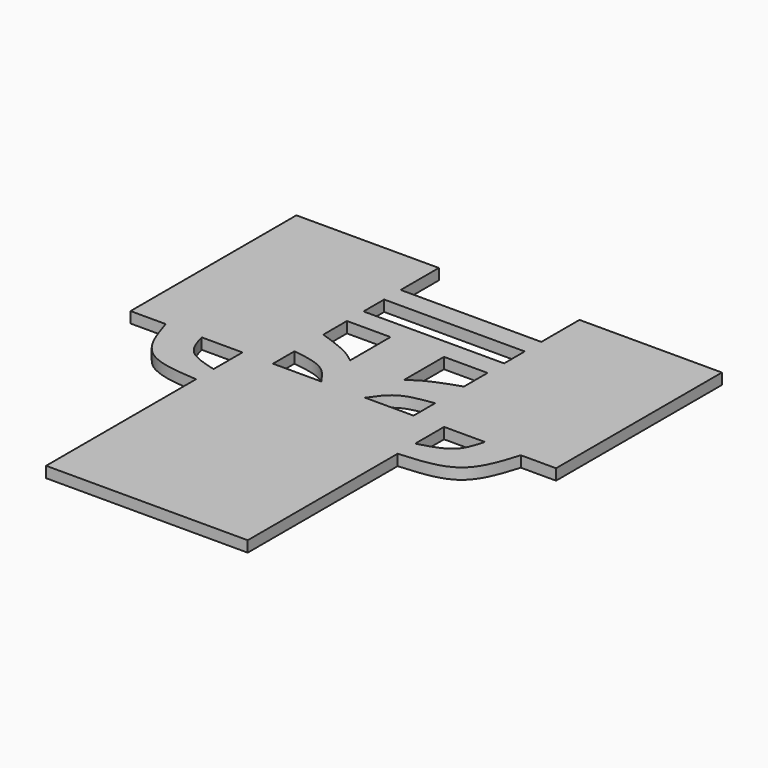
from build123d import *

# Parameters (mm, degrees)
F0_W     = 40.7416
F0_H     = 5.9913918376
F1_DEPTH = 3.175


# Not quite as in the source:
# - a feature names something its author has since deleted; it is built from what else it names


with BuildPart() as f1:
    # F0 (on Top) → F1 (new body)
    with BuildSketch(Plane.XY):
        Polygon((6.35, 2.420714612), (0, 2.420714612), (-6.35, 2.420714612), (-20.3708, 2.420714612), (-22.9107162118, 2.420714612), (-29.21, 2.420714612), (-29.21, -8.0478828564), (-29.21, -14.3978828564), (-29.21, -68.699285388), (29.21, -68.699285388), (29.21, -14.3978828564), (29.21, -8.0478828564), (29.21, 2.420714612), (20.3708, 2.420714612), align=None)
        Polygon((20.3708, 10.1967882365), (20.3708, 2.420714612), (29.21, 2.420714612), (41.0083, 2.420714612), (51.4477, 2.420714612), (61.6458, 2.420714612), (61.6458, 62.491714612), (20.3708, 62.491714612), (20.3708, 48.6805066466), (20.3708, 42.689114809), (20.3708, 35.2035965675), (20.3708, 29.2091965675), (20.3708, 20.6410996616), align=None)
        Polygon((-22.9107162118, 2.420714612), (-20.3708, 2.420714612), (-20.3708, 10.1967882365), (-20.3708, 20.6410996616), (-20.3708, 29.2091965675), (-20.3708, 35.2035965675), (-20.3708, 42.689114809), (-20.3708, 48.6805066466), (-20.3708, 62.491714612), (-61.6458, 62.491714612), (-61.6458, 2.420714612), (-51.4477, 2.420714612), (-41.0083, 2.420714612), (-29.21, 2.420714612), align=None)
        with BuildLine():
            add(Edge.make_bspline(
                [(29.21, -8.0478828564), (32.5638420451, -7.1347003919), (38.8822247108, -5.4143342635), (40.3293289084, -0.0814412218), (41.0083, 2.420714612)],
                knots=[0, 0, 0, 0, 0.5308070471, 1, 1, 1, 1], degree=3))
            Line((29.21, -8.0478828564), (29.21, -14.3978828564))
            add(Edge.make_bspline(
                [(29.21, -14.3978828564), (35.0623442189, -14.0006727781), (46.562333527, -13.2201459527), (49.8386841247, -2.7306682151), (51.4477, 2.420714612)],
                knots=[0, 0, 0, 0, 0.5088999704, 1, 1, 1, 1], degree=3))
            Line((51.4477, 2.420714612), (41.0083, 2.420714612))
        make_face()
        with BuildLine():
            Line((-29.21, -14.3978828564), (-29.21, -8.0478828564))
            add(Edge.make_bspline(
                [(-29.21, -8.0478828564), (-32.5638420451, -7.1347003919), (-38.8822247108, -5.4143342635), (-40.3293289084, -0.0814412218), (-41.0083, 2.420714612)],
                knots=[0, 0, 0, 0, 0.5308070471, 1, 1, 1, 1], degree=3))
            Line((-41.0083, 2.420714612), (-51.4477, 2.420714612))
            add(Edge.make_bspline(
                [(-29.21, -14.3978828564), (-35.0623442189, -14.0006727781), (-46.562333527, -13.2201459527), (-49.8386841247, -2.7306682151), (-51.4477, 2.420714612)],
                knots=[0, 0, 0, 0, 0.5088999704, 1, 1, 1, 1], degree=3))
        make_face()
        with Locations((0, 45.6848107278)):
            Rectangle(F0_W, F0_H)
        with BuildLine():
            Line((-6.35, 2.420714612), (0, 2.420714612))
            add(Edge.make_bspline(
                [(0, 2.420714612), (-2.1599363926, 6.9765171348), (-4.3198727852, 11.5323196577), (-7.7523121432, 14.5766604692)],
                knots=[0, 0, 0, 0, 0.5036722623, 0.5036722623, 0.5036722623, 0.5036722623], degree=3))
            add(Edge.make_bspline(
                [(-7.7523121432, 14.5766604692), (-11.1346998365, 17.5766088502), (-15.7527499182, 19.1088542559), (-20.3708, 20.6410996616)],
                knots=[0.5036722623, 0.5036722623, 0.5036722623, 0.5036722623, 1, 1, 1, 1], degree=3))
            Line((-20.3708, 20.6410996616), (-20.3708, 10.1967882365))
            add(Edge.make_bspline(
                [(-6.35, 2.420714612), (-7.7523121432, 4.4872624945), (-10.7420432518, 8.8931449662), (-17.0314139567, 9.7446667159), (-20.3708, 10.1967882365)],
                knots=[0, 0, 0, 0, 0.4690428979, 1, 1, 1, 1], degree=3))
        make_face()
        with BuildLine():
            add(Edge.make_bspline(
                [(0, 2.420714612), (2.1599363926, 6.9765171348), (4.3198727852, 11.5323196577), (7.7523121432, 14.5766604692)],
                knots=[0, 0, 0, 0, 0.5036722623, 0.5036722623, 0.5036722623, 0.5036722623], degree=3))
            Line((0, 2.420714612), (6.35, 2.420714612))
            add(Edge.make_bspline(
                [(6.35, 2.420714612), (7.7523121432, 4.4872624945), (10.7420432518, 8.8931449662), (17.0314139567, 9.7446667159), (20.3708, 10.1967882365)],
                knots=[0, 0, 0, 0, 0.4690428979, 1, 1, 1, 1], degree=3))
            Line((20.3708, 10.1967882365), (20.3708, 20.6410996616))
            add(Edge.make_bspline(
                [(7.7523121432, 14.5766604692), (11.1346998365, 17.5766088502), (15.7527499182, 19.1088542559), (20.3708, 20.6410996616)],
                knots=[0.5036722623, 0.5036722623, 0.5036722623, 0.5036722623, 1, 1, 1, 1], degree=3))
        make_face()
        with BuildLine():
            add(Edge.make_bspline(
                [(0, 2.420714612), (-2.1599363926, 6.9765171348), (-4.3198727852, 11.5323196577), (-7.7523121432, 14.5766604692)],
                knots=[0, 0, 0, 0, 0.5036722623, 0.5036722623, 0.5036722623, 0.5036722623], degree=3))
            add(Edge.make_bspline(
                [(0, 2.420714612), (2.1599363926, 6.9765171348), (4.3198727852, 11.5323196577), (7.7523121432, 14.5766604692)],
                knots=[0, 0, 0, 0, 0.5036722623, 0.5036722623, 0.5036722623, 0.5036722623], degree=3))
            Line((7.7523121432, 14.5766604692), (7.7523121432, 29.2091965675))
            Line((7.7523121432, 29.2091965675), (-7.7523121432, 29.2091965675))
            Line((-7.7523121432, 29.2091965675), (-7.7523121432, 14.5766604692))
        make_face()
        Polygon((-7.7523121432, 29.2091965675), (7.7523121432, 29.2091965675), (20.3708, 29.2091965675), (20.3708, 35.2035965675), (-20.3708, 35.2035965675), (-20.3708, 29.2091965675), align=None)
    extrude(amount=F1_DEPTH)


solid = f1.part
